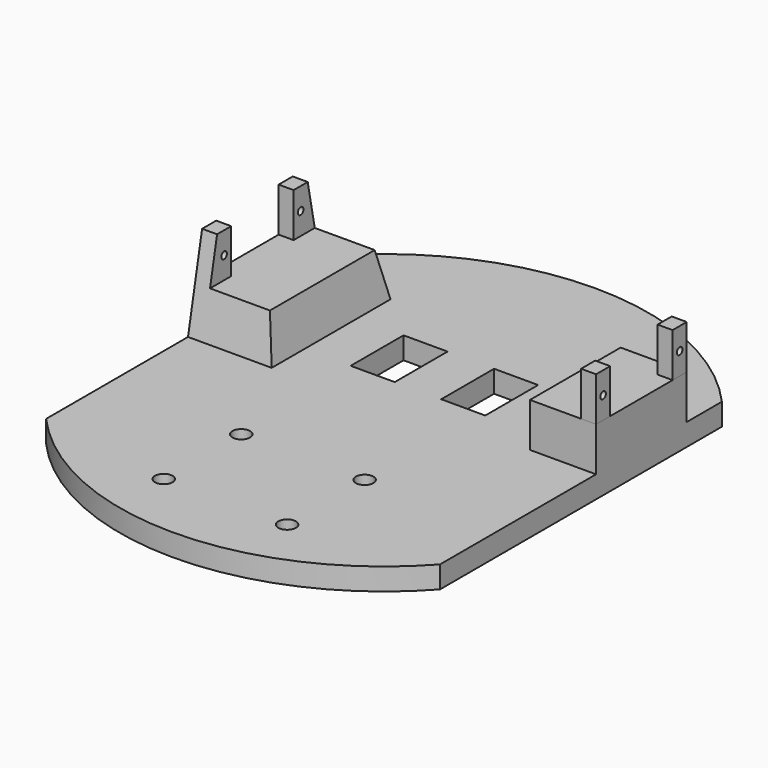
from build123d import *

# Parameters (mm, degrees)
F1_DEPTH      = 19.05
F2_W          = 4.318
F2_H          = 5.08
F3_DEPTH      = 12.7
F5_DEPTH      = 12.7
F7_D          = 5.08
F9_D          = 2.032
F10_W         = 12.7
F10_H         = 19.05
F11_DEPTH     = 19.051
F12_T4_DEPTH  = 85.0425549919
F12_T10_DEPTH = 85.0425549919
F12_T17_DEPTH = 85.0425549919
F12_T25_DEPTH = 85.0425549919
F12_T33_DEPTH = 32.6644
F12_T38_DEPTH = 85.0425712574
F12_T45_DEPTH = 85.0425712574
F12_T52_DEPTH = 85.0425712574
F12_T60_DEPTH = 85.0425712574
F12_T67_DEPTH = 98.6569549919
F12_T72_DEPTH = 151.0351099839
F12_T80_DEPTH = 151.0351262494
F12_T85_DEPTH = 98.6569549919
F12_S86_R     = 76.2
F12_T87_DEPTH = 53


# Not quite as in the source:
# - a fillet or chamfer that OpenCascade refuses, or shapes differently, is made with other operations: its cross-section is extruded or revolved along the edge and cut away or added


with BuildPart() as f1:
    # F0 (on Top) → F1 (new body)
    with BuildSketch(Plane.XY):
        with BuildLine():
            Line((56.7961519247, -50.7999717179), (56.7961013322, 50.8000282821))
            ThreePointArc((56.7961013322, 50.8000282821), (-3.79444e-05, 76.2), (-56.7961519247, 50.7999717179))
            Line((-56.7961519247, 50.7999717179), (-56.7961013322, -50.8000282821))
            ThreePointArc((-56.7961013322, -50.8000282821), (3.79444e-05, -76.2), (56.7961519247, -50.7999717179))
        make_face()
    extrude(amount=F1_DEPTH)

    # F2 (on face) → F3 (join)
    with BuildSketch(Plane.XY.offset(19.05)):
        with Locations((-54.6371318648, 35.56)):
            Rectangle(F2_W, F2_H)
        with Locations((-54.6371318648, 7.9756)):
            Rectangle(F2_W, F2_H)
        Polygon((56.7960989797, 33.0200565641), (56.7960939204, 38.1000565641), (52.4780939204, 38.1000522638), (52.4780989797, 33.0200522638), align=None)
        Polygon((56.7961264514, 5.4356565641), (56.7961213921, 10.5156565641), (52.4781213922, 10.5156522638), (52.4781264514, 5.4356522638), align=None)
    extrude(amount=F3_DEPTH)

    # F4 (on face) → F5 (cut)
    with BuildSketch(Plane.XY.offset(19.05)):
        with BuildLine():
            Line((-56.7961293352, 5.4356), (-56.7961013322, -50.8000282821))
            ThreePointArc((-56.7961013322, -50.8000282821), (3.79444e-05, -76.2), (56.7961519247, -50.7999717179))
            Line((56.7961519247, -50.7999717179), (56.7961239218, 5.4356565641))
            Line((56.7961239218, 5.4356565641), (52.4781264514, 5.4356565641))
            Line((52.4781264514, 5.4356565641), (37.7461239218, 5.4356565641))
            Line((37.7461239218, 5.4356565641), (37.7461239218, 38.1000565641))
            Line((37.7461239218, 38.1000565641), (52.4780939204, 38.1000565641))
            Line((52.4780939204, 38.1000565641), (56.7961076563, 38.1000565641))
            Line((56.7961076563, 38.1000565641), (56.7961013322, 50.8000282821))
            ThreePointArc((56.7961013322, 50.8000282821), (-3.79444e-05, 76.2), (-56.7961519247, 50.7999717179))
            Line((-56.7961519247, 50.7999717179), (-56.7961456007, 38.1))
            Line((-56.7961456007, 38.1), (-52.4781318648, 38.1))
            Line((-52.4781318648, 38.1), (-37.7461293352, 38.1))
            Line((-37.7461293352, 38.1), (-37.7461293352, 5.4356))
            Line((-37.7461293352, 5.4356), (-52.4781318648, 5.4356))
            Line((-52.4781318648, 5.4356), (-56.7961293352, 5.4356))
        make_face()
    extrude(amount=-F5_DEPTH, mode=Mode.SUBTRACT)

    # F7 (through all)
    with Locations(Plane.XY.offset(6.35)):
        with Locations((-17.78, -29.21), (17.78, -29.21), (17.78, -57.15), (-17.78, -57.15)):
            Hole(F7_D / 2)

    # F9 (through all)
    with Locations(Plane(origin=(-56.7961266285, -2.82821e-05, 0), x_dir=(4.98e-07, -1, 0), z_dir=(-1, -4.98e-07, 0))):
        with Locations((-35.5600282821, 25.4), (-7.9756282821, 25.4)):
            Hole(F9_D / 2)

    # F10 (on face) → F11 (cut, through all)
    with BuildSketch(Plane.XY.offset(19.05)):
        with Locations((13.0538625321, 21.7678)):
            Rectangle(F10_W, F10_H)
        with Locations((-13.0538625321, 21.7678)):
            Rectangle(F10_W, F10_H)
    extrude(amount=-F11_DEPTH, mode=Mode.SUBTRACT)

    # F12: chamfer of 5.08 x 25.4 on 3 edges, made by hand


with BuildPart() as f12_tool2:
    # F12_s3 → F12_t4 (new body)
    with BuildSketch(Plane.YZ.offset(-37.7461293352)):
        with BuildLine():
            Line((0.1563460067, 5.3537300335), (5.6348539933, 32.7462699665))
            Line((5.6348539933, 32.7462699665), (6.1428539933, 32.7462699665))
            ThreePointArc((6.1428539933, 32.7462699665), (5.9436, 19.5481349833), (5.9436, 6.35))
            Line((5.9436, 6.35), (5.4356, 5.842))
            ThreePointArc((5.4356, 5.842), (2.7959730033, 5.842), (0.1563460067, 4.8457300335))
            Line((0.1563460067, 4.8457300335), (0.1563460067, 5.3537300335))
        make_face()
    extrude(amount=-F12_T4_DEPTH)

    split(bisect_by=Plane.XY.offset(19.05), keep=Keep.BOTTOM)

    split(bisect_by=Plane.YZ.offset(-52.4781318648), keep=Keep.TOP)


with BuildPart() as f1_1:
    add(f1.part)

    # F12_t1: union F12_tool2
    add(f12_tool2.part)


with BuildPart() as f12_tool8:
    # F12_s9 → F12_t10 (new body)
    with BuildSketch(Plane.YZ.offset(-37.7461293352)):
        with BuildLine():
            Line((0.1563460067, 5.3537300335), (5.6348539933, 32.7462699665))
            Line((5.6348539933, 32.7462699665), (6.1428539933, 32.7462699665))
            ThreePointArc((6.1428539933, 32.7462699665), (5.9436, 19.5481349833), (5.9436, 6.35))
            Line((5.9436, 6.35), (5.4356, 5.842))
            ThreePointArc((5.4356, 5.842), (2.7959730033, 5.842), (0.1563460067, 4.8457300335))
            Line((0.1563460067, 4.8457300335), (0.1563460067, 5.3537300335))
        make_face()
    extrude(amount=-F12_T10_DEPTH)

    split(bisect_by=Plane.YZ.offset(-56.7961318648), keep=Keep.TOP)

    split(bisect_by=Plane.XY.offset(19.05), keep=Keep.BOTTOM)

    split(bisect_by=Plane.YZ.offset(-52.4781318648), keep=Keep.BOTTOM)


with BuildPart() as f1_2:
    add(f1_1.part)

    # F12_t7: union F12_tool8
    add(f12_tool8.part)


with BuildPart() as f12_tool15:
    # F12_s16 → F12_t17 (new body)
    with BuildSketch(Plane.YZ.offset(-37.7461293352)):
        with BuildLine():
            Line((0.1563460067, 5.3537300335), (5.6348539933, 32.7462699665))
            Line((5.6348539933, 32.7462699665), (6.1428539933, 32.7462699665))
            ThreePointArc((6.1428539933, 32.7462699665), (5.9436, 19.5481349833), (5.9436, 6.35))
            Line((5.9436, 6.35), (5.4356, 5.842))
            ThreePointArc((5.4356, 5.842), (2.7959730033, 5.842), (0.1563460067, 4.8457300335))
            Line((0.1563460067, 4.8457300335), (0.1563460067, 5.3537300335))
        make_face()
    extrude(amount=-F12_T17_DEPTH)

    split(bisect_by=Plane.YZ.offset(-56.7961318648), keep=Keep.TOP)

    split(bisect_by=Plane.XY.offset(19.05), keep=Keep.TOP)

    split(bisect_by=Plane.YZ.offset(-52.4781318648), keep=Keep.BOTTOM)

    split(bisect_by=Plane.XY.offset(31.75), keep=Keep.BOTTOM)


with BuildPart() as f1_3:
    add(f1_2.part)

    # F12_t14: union F12_tool15
    add(f12_tool15.part)


with BuildPart() as f12_tool23:
    # F12_s24 → F12_t25 (new body)
    with BuildSketch(Plane.YZ.offset(-37.7461293352)):
        with BuildLine():
            Line((0.1563460067, 5.3537300335), (5.6348539933, 32.7462699665))
            Line((5.6348539933, 32.7462699665), (6.1428539933, 32.7462699665))
            ThreePointArc((6.1428539933, 32.7462699665), (5.9436, 19.5481349833), (5.9436, 6.35))
            Line((5.9436, 6.35), (5.4356, 5.842))
            ThreePointArc((5.4356, 5.842), (2.7959730033, 5.842), (0.1563460067, 4.8457300335))
            Line((0.1563460067, 4.8457300335), (0.1563460067, 5.3537300335))
        make_face()
    extrude(amount=-F12_T25_DEPTH)

    split(bisect_by=Plane.YZ.offset(-56.7961293352), keep=Keep.BOTTOM)

    split(bisect_by=Plane.YZ.offset(-56.7961318648), keep=Keep.TOP)

    split(bisect_by=Plane.XY.offset(19.05), keep=Keep.TOP)

    split(bisect_by=Plane.XY.offset(31.75), keep=Keep.BOTTOM)


with BuildPart() as f1_4:
    add(f1_3.part)

    # F12_t22: union F12_tool23
    add(f12_tool23.part)


with BuildPart() as f12_tool31:
    # F12_s32 → F12_t33 (new body)
    with BuildSketch(Plane.XZ.offset(-38.1)):
        with BuildLine():
            Line((-32.4668753419, 5.3537300335), (-37.9453833285, 32.7462699665))
            Line((-37.9453833285, 32.7462699665), (-38.4533833285, 32.7462699665))
            ThreePointArc((-38.4533833285, 32.7462699665), (-38.2541293352, 19.5481349833), (-38.2541293352, 6.35))
            Line((-38.2541293352, 6.35), (-37.7461293352, 5.842))
            ThreePointArc((-37.7461293352, 5.842), (-35.1065023386, 5.842), (-32.4668753419, 4.8457300335))
            Line((-32.4668753419, 4.8457300335), (-32.4668753419, 5.3537300335))
        make_face()
    extrude(amount=F12_T33_DEPTH)

    split(bisect_by=Plane.XY.offset(19.05), keep=Keep.BOTTOM)


with BuildPart() as f1_5:
    add(f1_4.part)

    # F12_t30: union F12_tool31
    add(f12_tool31.part)


with BuildPart() as f12_tool36:
    # F12_s37 → F12_t38 (new body)
    with BuildSketch(Plane.YZ.offset(-122.7887005926)):
        with BuildLine():
            Line((43.3792539933, 5.3537300335), (37.9007460067, 32.7462699665))
            Line((37.9007460067, 32.7462699665), (37.3927460067, 32.7462699665))
            ThreePointArc((37.3927460067, 32.7462699665), (37.592, 19.5481349833), (37.592, 6.35))
            Line((37.592, 6.35), (38.1, 5.842))
            ThreePointArc((38.1, 5.842), (40.7396269967, 5.842), (43.3792539933, 4.8457300335))
            Line((43.3792539933, 4.8457300335), (43.3792539933, 5.3537300335))
        make_face()
    extrude(amount=F12_T38_DEPTH)

    split(bisect_by=Plane.YZ.offset(-56.7961456007), keep=Keep.TOP)

    split(bisect_by=Plane.XY.offset(19.05), keep=Keep.BOTTOM)

    split(bisect_by=Plane.YZ.offset(-56.7961318648), keep=Keep.BOTTOM)


with BuildPart() as f1_6:
    add(f1_5.part)

    # F12_t35: union F12_tool36
    add(f12_tool36.part)


with BuildPart() as f12_tool43:
    # F12_s44 → F12_t45 (new body)
    with BuildSketch(Plane.YZ.offset(-122.7887005926)):
        with BuildLine():
            Line((43.3792539933, 5.3537300335), (37.9007460067, 32.7462699665))
            Line((37.9007460067, 32.7462699665), (37.3927460067, 32.7462699665))
            ThreePointArc((37.3927460067, 32.7462699665), (37.592, 19.5481349833), (37.592, 6.35))
            Line((37.592, 6.35), (38.1, 5.842))
            ThreePointArc((38.1, 5.842), (40.7396269967, 5.842), (43.3792539933, 4.8457300335))
            Line((43.3792539933, 4.8457300335), (43.3792539933, 5.3537300335))
        make_face()
    extrude(amount=F12_T45_DEPTH)

    split(bisect_by=Plane.XY.offset(19.05), keep=Keep.BOTTOM)

    split(bisect_by=Plane.YZ.offset(-56.7961318648), keep=Keep.TOP)

    split(bisect_by=Plane.YZ.offset(-52.4781318648), keep=Keep.BOTTOM)


with BuildPart() as f1_7:
    add(f1_6.part)

    # F12_t42: union F12_tool43
    add(f12_tool43.part)


with BuildPart() as f12_tool50:
    # F12_s51 → F12_t52 (new body)
    with BuildSketch(Plane.YZ.offset(-122.7887005926)):
        with BuildLine():
            Line((43.3792539933, 5.3537300335), (37.9007460067, 32.7462699665))
            Line((37.9007460067, 32.7462699665), (37.3927460067, 32.7462699665))
            ThreePointArc((37.3927460067, 32.7462699665), (37.592, 19.5481349833), (37.592, 6.35))
            Line((37.592, 6.35), (38.1, 5.842))
            ThreePointArc((38.1, 5.842), (40.7396269967, 5.842), (43.3792539933, 4.8457300335))
            Line((43.3792539933, 4.8457300335), (43.3792539933, 5.3537300335))
        make_face()
    extrude(amount=F12_T52_DEPTH)

    split(bisect_by=Plane.XY.offset(19.05), keep=Keep.TOP)

    split(bisect_by=Plane.YZ.offset(-56.7961318648), keep=Keep.TOP)

    split(bisect_by=Plane.YZ.offset(-52.4781318648), keep=Keep.BOTTOM)

    split(bisect_by=Plane.XY.offset(31.75), keep=Keep.BOTTOM)


with BuildPart() as f1_8:
    add(f1_7.part)

    # F12_t49: union F12_tool50
    add(f12_tool50.part)


with BuildPart() as f12_tool58:
    # F12_s59 → F12_t60 (new body)
    with BuildSketch(Plane.YZ.offset(-122.7887005926)):
        with BuildLine():
            Line((43.3792539933, 5.3537300335), (37.9007460067, 32.7462699665))
            Line((37.9007460067, 32.7462699665), (37.3927460067, 32.7462699665))
            ThreePointArc((37.3927460067, 32.7462699665), (37.592, 19.5481349833), (37.592, 6.35))
            Line((37.592, 6.35), (38.1, 5.842))
            ThreePointArc((38.1, 5.842), (40.7396269967, 5.842), (43.3792539933, 4.8457300335))
            Line((43.3792539933, 4.8457300335), (43.3792539933, 5.3537300335))
        make_face()
    extrude(amount=F12_T60_DEPTH)

    split(bisect_by=Plane.XY.offset(19.05), keep=Keep.BOTTOM)

    split(bisect_by=Plane.YZ.offset(-52.4781318648), keep=Keep.TOP)


with BuildPart() as f1_9:
    add(f1_8.part)

    # F12_t57: union F12_tool58
    add(f12_tool58.part)


with BuildPart() as f12_tool65:
    # F12_s66 → F12_t67 (new body)
    with BuildSketch(Plane.XZ.offset(-38.1)):
        with BuildLine():
            Line((-32.4668753419, 5.3537300335), (-37.9453833285, 32.7462699665))
            Line((-37.9453833285, 32.7462699665), (-38.4533833285, 32.7462699665))
            ThreePointArc((-38.4533833285, 32.7462699665), (-38.2541293352, 19.5481349833), (-38.2541293352, 6.35))
            Line((-38.2541293352, 6.35), (-37.7461293352, 5.842))
            ThreePointArc((-37.7461293352, 5.842), (-35.1065023386, 5.842), (-32.4668753419, 4.8457300335))
            Line((-32.4668753419, 4.8457300335), (-32.4668753419, 5.3537300335))
        make_face()
    extrude(amount=F12_T67_DEPTH)

    split(bisect_by=Plane.XZ.offset(-5.4356), keep=Keep.TOP)

    split(bisect_by=Plane.XY.offset(19.05), keep=Keep.BOTTOM)


with BuildPart() as f12_tool70:
    # F12_s71 → F12_t72 (new body)
    with BuildSketch(Plane.YZ.offset(28.2464256567)):
        with BuildLine():
            Line((0.1563460067, 5.3537300335), (5.6348539933, 32.7462699665))
            Line((5.6348539933, 32.7462699665), (6.1428539933, 32.7462699665))
            ThreePointArc((6.1428539933, 32.7462699665), (5.9436, 19.5481349833), (5.9436, 6.35))
            Line((5.9436, 6.35), (5.4356, 5.842))
            ThreePointArc((5.4356, 5.842), (2.7959730033, 5.842), (0.1563460067, 4.8457300335))
            Line((0.1563460067, 4.8457300335), (0.1563460067, 5.3537300335))
        make_face()
    extrude(amount=-F12_T72_DEPTH)

    split(bisect_by=Plane.YZ.offset(-37.7461293352), keep=Keep.TOP)

    split(bisect_by=Plane.XY.offset(19.05), keep=Keep.BOTTOM)


with BuildPart() as f12_tool65_1:
    add(f12_tool65.part)

    # F12_t75: intersect F12_tool70
    add(f12_tool70.part, mode=Mode.INTERSECT)


with BuildPart() as f1_10:
    add(f1_9.part)

    # F12_t63: union F12_tool65
    add(f12_tool65_1.part)


with BuildPart() as f12_tool78:
    # F12_s79 → F12_t80 (new body)
    with BuildSketch(Plane.YZ.offset(-122.7887005926)):
        with BuildLine():
            Line((43.3792539933, 5.3537300335), (37.9007460067, 32.7462699665))
            Line((37.9007460067, 32.7462699665), (37.3927460067, 32.7462699665))
            ThreePointArc((37.3927460067, 32.7462699665), (37.592, 19.5481349833), (37.592, 6.35))
            Line((37.592, 6.35), (38.1, 5.842))
            ThreePointArc((38.1, 5.842), (40.7396269967, 5.842), (43.3792539933, 4.8457300335))
            Line((43.3792539933, 4.8457300335), (43.3792539933, 5.3537300335))
        make_face()
    extrude(amount=F12_T80_DEPTH)

    split(bisect_by=Plane.XY.offset(19.05), keep=Keep.BOTTOM)

    split(bisect_by=Plane.YZ.offset(-37.7461293352), keep=Keep.TOP)


with BuildPart() as f12_tool83:
    # F12_s84 → F12_t85 (new body)
    with BuildSketch(Plane.XZ.offset(-104.0925549919)):
        with BuildLine():
            Line((-32.4668753419, 5.3537300335), (-37.9453833285, 32.7462699665))
            Line((-37.9453833285, 32.7462699665), (-38.4533833285, 32.7462699665))
            ThreePointArc((-38.4533833285, 32.7462699665), (-38.2541293352, 19.5481349833), (-38.2541293352, 6.35))
            Line((-38.2541293352, 6.35), (-37.7461293352, 5.842))
            ThreePointArc((-37.7461293352, 5.842), (-35.1065023386, 5.842), (-32.4668753419, 4.8457300335))
            Line((-32.4668753419, 4.8457300335), (-32.4668753419, 5.3537300335))
        make_face()
    extrude(amount=F12_T85_DEPTH)

    # F12_s86 → F12_t87 (intersect, symmetric)
    with BuildSketch(Plane.XY.offset(18.8)):
        Circle(F12_S86_R)
    extrude(amount=F12_T87_DEPTH, both=True, mode=Mode.INTERSECT)

    split(bisect_by=Plane.XY.offset(19.05), keep=Keep.BOTTOM)

    split(bisect_by=Plane.XZ.offset(-38.1), keep=Keep.BOTTOM)


with BuildPart() as f12_tool78_1:
    add(f12_tool78.part)

    # F12_t90: intersect F12_tool83
    add(f12_tool83.part, mode=Mode.INTERSECT)


with BuildPart() as f1_11:
    add(f1_10.part)

    # F12_t76: union F12_tool78
    add(f12_tool78_1.part)


solid = f1_11.part
